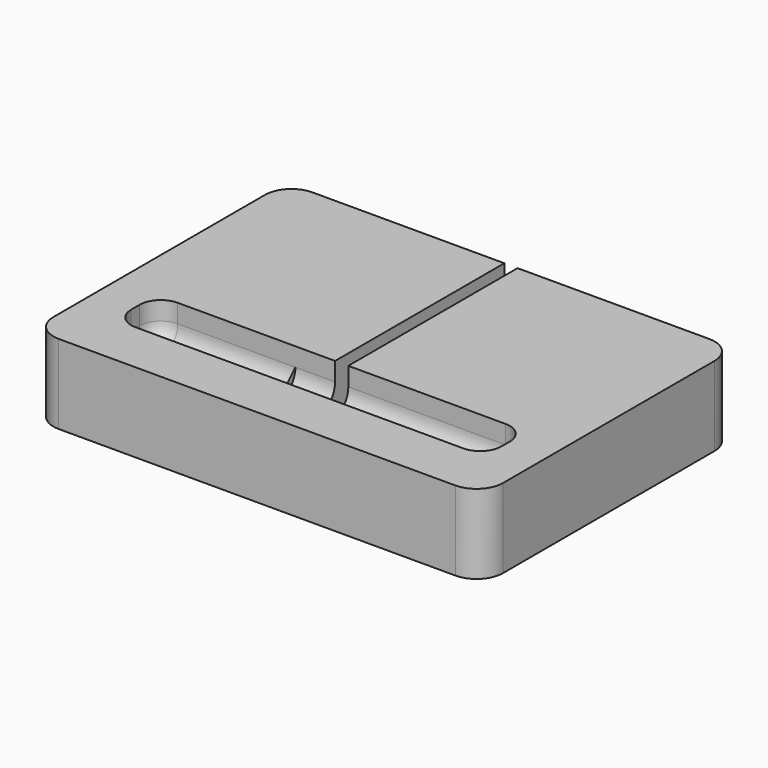
from build123d import *

# Parameters (mm, degrees)
F0_W         = 107.95
F0_H         = 76.2
F1_DEPTH     = 19.05
F2_W         = 3.175
F2_H         = 63.5
F3_DEPTH     = 19.051
F4_W         = 42.8625
F4_H         = 12.7
F5_DEPTH     = 9.525
F7_DEPTH     = 12.7
F8_R         = 5.08
F9_T1_DEPTH  = 2.54
F9_T6_DEPTH  = 37.7825
F9_S7_R      = 3.175
F9_T8_DEPTH  = 21
F9_T12_DEPTH = 50.4825
F9_S14_R     = 3.175
F9_T15_DEPTH = 27
F9_T17_ANGLE = 90
F9_T19_ANGLE = 90
F9_T23_DEPTH = 50.4825
F9_S25_R     = 3.175
F9_T26_DEPTH = 27
F9_T30_DEPTH = 37.7825
F9_S31_R     = 3.175
F9_T32_DEPTH = 21
F10_R        = 5.08
F11_R        = 6.35


# Not quite as in the source:
# - a fillet or chamfer that OpenCascade refuses, or shapes differently, is made with other operations: its cross-section is extruded or revolved along the edge and cut away or added


with BuildPart() as f1:
    # F0 (on Top) → F1 (new body)
    with BuildSketch(Plane.XY):
        Rectangle(F0_W, F0_H)
    extrude(amount=-F1_DEPTH)

    # F2 (on face) → F3 (cut, through all)
    with BuildSketch(Plane.XY):
        with Locations((0, 6.35)):
            Rectangle(F2_W, F2_H)
    extrude(amount=-F3_DEPTH, mode=Mode.SUBTRACT)

    # F4 (on face) → F5 (cut)
    with BuildSketch(Plane.XY):
        with Locations((23.01875, -19.05)):
            Rectangle(F4_W, F4_H)
        with Locations((-23.01875, -19.05)):
            Rectangle(F4_W, F4_H)
    extrude(amount=-F5_DEPTH, mode=Mode.SUBTRACT)

    # F6 (on face) → F7 (cut)
    with BuildSketch(Plane.XY.offset(-9.525)):
        with BuildLine():
            Line((1.5875, -15.875), (-1.5875, -15.875))
            ThreePointArc((-1.5875, -15.875), (-3.8325640303, -16.8049359697), (-4.7625, -19.05))
            ThreePointArc((-4.7625, -19.05), (-3.8325640303, -21.2950640303), (-1.5875, -22.225))
            Line((-1.5875, -22.225), (1.5875, -22.225))
            Line((1.5875, -22.225), (1.5875, -15.875))
        make_face()
        with BuildLine():
            ThreePointArc((4.7625, -19.05), (3.8325640303, -16.8049359697), (1.5875, -15.875))
            Line((1.5875, -15.875), (1.5875, -22.225))
            ThreePointArc((1.5875, -22.225), (3.8325640303, -21.2950640303), (4.7625, -19.05))
        make_face()
    extrude(amount=-F7_DEPTH, mode=Mode.SUBTRACT)

    # F8
    f8_edges = [f1.edges().sort_by_distance(p)[0] for p in [
        (-44.45, -12.7, -4.7625),
        (-44.45, -25.4, -4.7625),
        (44.45, -12.7, -4.7625),
        (44.45, -25.4, -4.7625),
    ]]
    fillet(f8_edges, radius=F8_R)

    # F9: fillet of radius 5.08 on 1 edges, made by hand

    # F9_s2 → F9_t1 (join)
    with BuildSketch(Plane.XZ.offset(17.78)):
        with BuildLine():
            ThreePointArc((44.45, -4.445), (42.9621024484, -8.0371024484), (39.37, -9.525))
            Line((39.37, -9.525), (44.45, -9.525))
            Line((44.45, -9.525), (44.45, -4.445))
        make_face()
    extrude(amount=F9_T1_DEPTH)


with BuildPart() as f9_tool4:
    # F9_s5 → F9_t6 (new body)
    with BuildSketch(Plane.YZ.offset(39.37)):
        with BuildLine():
            ThreePointArc((-12.7, -4.445), (-14.1878975516, -8.0371024484), (-17.78, -9.525))
            Line((-17.78, -9.525), (-12.7, -9.525))
            Line((-12.7, -9.525), (-12.7, -4.445))
        make_face()
    extrude(amount=-F9_T6_DEPTH)

    # F9_s7 → F9_t8 (cut, symmetric)
    with BuildSketch(Plane.XY.offset(-7)):
        with Locations((1.5875, -19.05)):
            Circle(F9_S7_R)
    extrude(amount=F9_T8_DEPTH, both=True, mode=Mode.SUBTRACT)


with BuildPart() as f1_1:
    add(f1.part)

    # F9_t3: union F9_tool4
    add(f9_tool4.part)


with BuildPart() as f9_tool10:
    # F9_s11 → F9_t12 (new body)
    with BuildSketch(Plane.YZ.offset(39.37)):
        with BuildLine():
            ThreePointArc((-12.7, -4.445), (-14.1878975516, -8.0371024484), (-17.78, -9.525))
            Line((-17.78, -9.525), (-12.7, -9.525))
            Line((-12.7, -9.525), (-12.7, -4.445))
        make_face()
    extrude(amount=-F9_T12_DEPTH)

    split(bisect_by=Plane.YZ.offset(-1.5875), keep=Keep.BOTTOM)

    # F9_s14 → F9_t15 (cut, symmetric)
    with BuildSketch(Plane.XY.offset(-7)):
        with Locations((-1.5875, -19.05)):
            Circle(F9_S14_R)
    extrude(amount=F9_T15_DEPTH, both=True, mode=Mode.SUBTRACT)


with BuildPart() as f1_2:
    add(f1_1.part)

    # F9_t9: union F9_tool10
    add(f9_tool10.part)

    # F9_s16 → F9_t17 (revolve)
    with BuildSketch(Plane.YZ.offset(39.37)):
        with BuildLine():
            ThreePointArc((-12.7, -4.445), (-14.1878975516, -8.0371024484), (-17.78, -9.525))
            Line((-17.78, -9.525), (-12.7, -9.525))
            Line((-12.7, -9.525), (-12.7, -4.445))
        make_face()
    revolve(axis=Axis((39.37, -17.78, -9.525), (0, 0, -1)), revolution_arc=F9_T17_ANGLE)

    # F9_s18 → F9_t19 (revolve)
    with BuildSketch(Plane.XZ.offset(20.32)):
        with BuildLine():
            ThreePointArc((44.45, -4.445), (42.9621024484, -8.0371024484), (39.37, -9.525))
            Line((39.37, -9.525), (44.45, -9.525))
            Line((44.45, -9.525), (44.45, -4.445))
        make_face()
    revolve(axis=Axis((39.37, -20.32, -9.525), (0, 0, -1)), revolution_arc=F9_T19_ANGLE)


with BuildPart() as f9_tool21:
    # F9_s22 → F9_t23 (new body)
    with BuildSketch(Plane.YZ.offset(-11.1125)):
        with BuildLine():
            ThreePointArc((-25.4, -4.445), (-23.9121024484, -8.0371024484), (-20.32, -9.525))
            Line((-20.32, -9.525), (-25.4, -9.525))
            Line((-25.4, -9.525), (-25.4, -4.445))
        make_face()
    extrude(amount=F9_T23_DEPTH)

    split(bisect_by=Plane.YZ.offset(-1.5875), keep=Keep.BOTTOM)

    # F9_s25 → F9_t26 (cut, symmetric)
    with BuildSketch(Plane.XY.offset(-7)):
        with Locations((-1.5875, -19.05)):
            Circle(F9_S25_R)
    extrude(amount=F9_T26_DEPTH, both=True, mode=Mode.SUBTRACT)


with BuildPart() as f1_3:
    add(f1_2.part)

    # F9_t20: union F9_tool21
    add(f9_tool21.part)


with BuildPart() as f9_tool28:
    # F9_s29 → F9_t30 (new body)
    with BuildSketch(Plane.YZ.offset(1.5875)):
        with BuildLine():
            ThreePointArc((-25.4, -4.445), (-23.9121024484, -8.0371024484), (-20.32, -9.525))
            Line((-20.32, -9.525), (-25.4, -9.525))
            Line((-25.4, -9.525), (-25.4, -4.445))
        make_face()
    extrude(amount=F9_T30_DEPTH)

    # F9_s31 → F9_t32 (cut, symmetric)
    with BuildSketch(Plane.XY.offset(-7)):
        with Locations((1.5875, -19.05)):
            Circle(F9_S31_R)
    extrude(amount=F9_T32_DEPTH, both=True, mode=Mode.SUBTRACT)


with BuildPart() as f1_4:
    add(f1_3.part)

    # F9_t27: union F9_tool28
    add(f9_tool28.part)

    # F10
    f10_edges = [f1_4.edges().sort_by_distance(p)[0] for p in [
        (-25.24125, -12.7, -9.525),
    ]]
    fillet(f10_edges, radius=F10_R)

    # F11
    f11_edges = [f1_4.edges().sort_by_distance(p)[0] for p in [
        (53.975, -38.1, -9.525),
        (53.975, 38.1, -9.525),
        (-53.975, -38.1, -9.525),
        (-53.975, 38.1, -9.525),
    ]]
    fillet(f11_edges, radius=F11_R)


solid = f1_4.part
